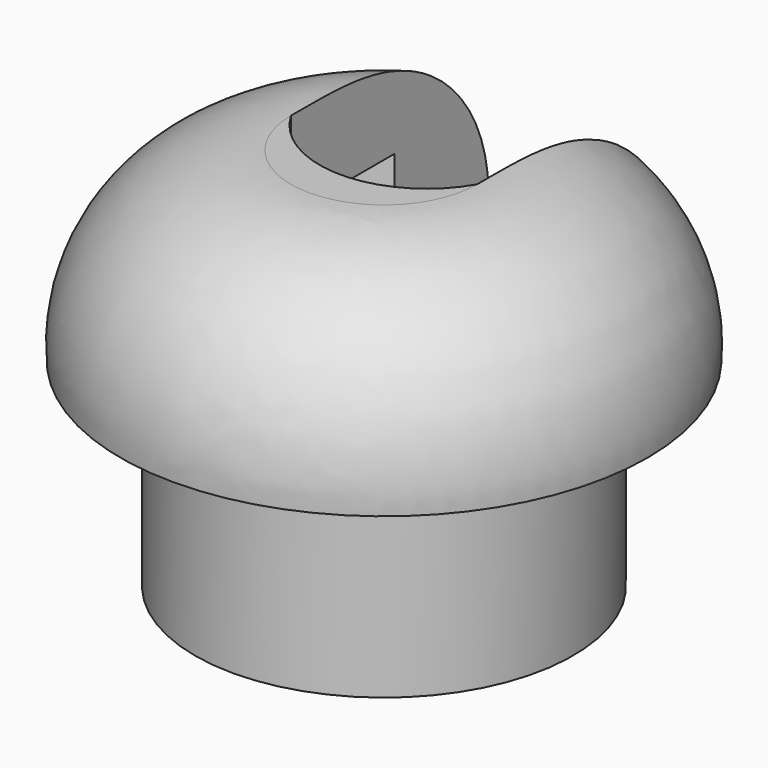
from build123d import *

# Parameters (mm, degrees)
F4_DEPTH = 15.4777297208
F6_DEPTH = 12


with BuildPart() as f2:
    # F1 (on Front) → F2 (revolve)
    with BuildSketch(Plane.XZ):
        with BuildLine():
            Line((0, 15.4767297208), (0, 0))
            Line((0, 0), (7.625, 0))
            Line((7.625, 0), (7.625, 8))
            Line((7.625, 8), (10.625, 8))
            ThreePointArc((10.625, 8), (8.8302197506, 13.2471744611), (3.752507735, 15.4767297208))
            Line((3.752507735, 15.4767297208), (0, 15.4767297208))
        make_face()
    revolve(axis=Axis((0, 0, 0), (0, 0, 1)))

    # F3 (on face) → F4 (cut, through all)
    with BuildSketch(Plane.XY.offset(15.4767297208)):
        with BuildLine():
            ThreePointArc((-3.752507735, 0), (0, -2.1712493207), (3.752507735, 0))
            ThreePointArc((3.752507735, 0), (0, 3.752507735), (-3.752507735, 0))
        make_face()
        with BuildLine():
            Line((3.752507735, 0), (3.752507735, 9.9402872543))
            ThreePointArc((3.752507735, 9.9402872543), (0, 10.625), (-3.752507735, 9.9402872543))
            Line((-3.752507735, 9.9402872543), (-3.752507735, 0))
            ThreePointArc((-3.752507735, 0), (0, 3.752507735), (3.752507735, 0))
        make_face()
        with BuildLine():
            ThreePointArc((-3.752507735, 9.9402872543), (0, 10.625), (3.752507735, 9.9402872543))
            Line((3.752507735, 9.9402872543), (3.752507735, 12.1829835698))
            Line((3.752507735, 12.1829835698), (-3.752507735, 12.1829835698))
            Line((-3.752507735, 12.1829835698), (-3.752507735, 9.9402872543))
        make_face()
    extrude(amount=-F4_DEPTH, mode=Mode.SUBTRACT)

    # F5 (on face) → F6 (cut)
    with BuildSketch(Plane(origin=(0, 0, 0), x_dir=(1, 0, 0), z_dir=(0, 0, -1))):
        with BuildLine():
            ThreePointArc((3.752507735, -5.21529584), (5.7179754808, -2.9300821492), (6.425, 0))
            ThreePointArc((6.425, 0), (-2.9300821492, 5.7179754808), (-3.752507735, -5.21529584))
            Line((-3.752507735, -5.21529584), (-3.752507735, 0))
            ThreePointArc((-3.752507735, 0), (0, 2.1712493207), (3.752507735, 0))
            Line((3.752507735, 0), (3.752507735, -5.21529584))
        make_face()
        with BuildLine():
            Line((-3.752507735, 0), (-3.752507735, -5.21529584))
            ThreePointArc((-3.752507735, -5.21529584), (0, -6.425), (3.752507735, -5.21529584))
            Line((3.752507735, -5.21529584), (3.752507735, 0))
            ThreePointArc((3.752507735, 0), (0, 2.1712493207), (-3.752507735, 0))
        make_face()
    extrude(amount=-F6_DEPTH, mode=Mode.SUBTRACT)


solid = f2.part
